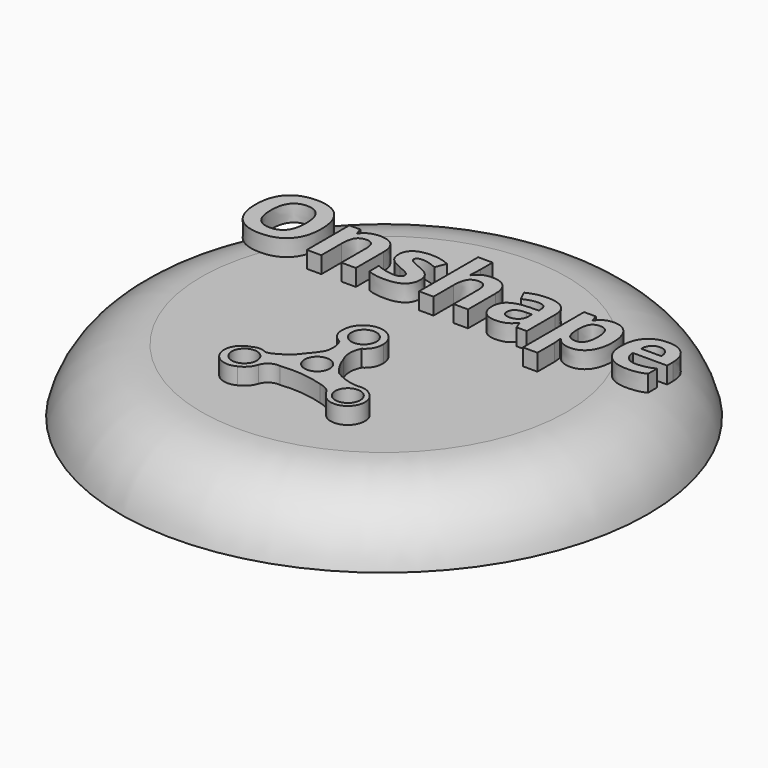
from build123d import *

# Parameters (mm, degrees)
F0_R         = 15.805
F1_DEPTH     = 3.81
F3_TEXT_SIZE = 5.8197312885
F4_DEPTH     = 1
F6_R         = 0.75
F7_DEPTH     = 1


# Not quite as in the source:
# - a fillet or chamfer that OpenCascade refuses, or shapes differently, is made with other operations: its cross-section is extruded or revolved along the edge and cut away or added
# - Text() gives the source's letters only with a copy of the font that has no kerning and outlines rounded to 1/6400 em; it was checked with that copy


with BuildPart() as f1:
    # F0 (on Top) → F1 (new body)
    with BuildSketch(Plane.XY):
        Circle(F0_R)
    extrude(amount=F1_DEPTH)

    # F2: fillet of radius 5 on 1 edges, made by hand

    # F2_s1 → F2_t2 (revolve, cut)
    with BuildSketch(Plane.XZ):
        with BuildLine():
            ThreePointArc((15.805, 0), (14.0349341008, 2.7438276526), (10.9486742284, 3.81))
            Line((10.9486742284, 3.81), (15.805, 3.81))
            Line((15.805, 3.81), (15.805, 0))
        make_face()
    revolve(axis=Axis((0, 0, 3.81), (0, 0, 1)), mode=Mode.SUBTRACT)

    # F3 (on face) → F4 (join)
    with BuildSketch(Plane.XY.offset(3.81)):
        with Locations((-12.6856137067, 3.719474189)):
            Text('Onshape', F3_TEXT_SIZE, font='Open Sans', font_style=FontStyle.BOLD, text_align=(TextAlign.LEFT, TextAlign.BOTTOM))
    extrude(amount=F4_DEPTH)

    # F6 (on face) → F7 (join)
    with BuildSketch(Plane.XY.offset(3.81)):
        with BuildLine():
            ThreePointArc((0.6517725415, -2.4959768634), (1.0496267958, -2.0753870693), (1.1650670785, -1.5080623617))
            ThreePointArc((1.1650670785, -1.5080623617), (-0.0326198642, -0.3425671333), (-1.230306807, -1.5080623617))
            ThreePointArc((-1.230306807, -1.5080623617), (-1.1063250132, -2.1233603441), (-0.6392406649, -2.5426398497))
            ThreePointArc((-0.6392406649, -2.5426398497), (-0.454048202, -3.1255160568), (-0.5286578089, -3.7325369194))
            ThreePointArc((-0.5286578089, -3.7325369194), (-0.8020989328, -4.1398712461), (-1.1165763717, -4.5164283365))
            ThreePointArc((-1.1165763717, -4.5164283365), (-1.5447835525, -5.0095430703), (-2.0964406431, -5.3591113538))
            ThreePointArc((-2.0964406431, -5.3591113538), (-2.3631101045, -5.5130095162), (-2.6647618506, -5.5746817961))
            ThreePointArc((-2.6647618506, -5.5746817961), (-3.0861033592, -5.455605353), (-3.5074448679, -5.5746817961))
            ThreePointArc((-3.5074448679, -5.5746817961), (-4.2369689218, -6.9676881184), (-2.7627481613, -7.5148125179))
            ThreePointArc((-2.7627481613, -7.5148125179), (-2.3440710579, -7.2189850446), (-2.0964406431, -6.7701158114))
            ThreePointArc((-2.0964406431, -6.7701158114), (-1.7679026827, -6.357753915), (-1.2537572766, -6.2409890816))
            ThreePointArc((-1.2537572766, -6.2409890816), (0.0722883441, -6.2340875096), (1.3722787844, -6.4957542345))
            ThreePointArc((1.3722787844, -6.4957542345), (1.6880765903, -6.6062751945), (1.9797945861, -6.7701158114))
            ThreePointArc((1.9797945861, -6.7701158114), (2.1665815655, -7.0510391049), (2.3717400618, -7.3188398965))
            ThreePointArc((2.3717400618, -7.3188398965), (3.9132771757, -7.2953405712), (3.6847579759, -5.7706544176))
            ThreePointArc((3.6847579759, -5.7706544176), (3.3163528533, -5.5785061448), (2.9008667916, -5.5746817961))
            ThreePointArc((2.9008667916, -5.5746817961), (2.1025476803, -5.4358737962), (1.3722787844, -5.0847493112))
            ThreePointArc((1.3722787844, -5.0847493112), (0.945670213, -4.5061587484), (0.6517725415, -3.8501205854))
            ThreePointArc((0.6517725415, -3.8501205854), (0.4894513603, -3.1730487244), (0.6517725415, -2.4959768634))
        make_face()
        with Locations((-3.1685938203, -6.4946736768)):
            Circle(F6_R, mode=Mode.SUBTRACT)
        with Locations((3.1130756933, -6.6076747296)):
            Circle(F6_R, mode=Mode.SUBTRACT)
        with Locations((0, -5.0080623617)):
            Circle(F6_R, mode=Mode.SUBTRACT)
        with Locations((0, -1.5080623617)):
            Circle(F6_R, mode=Mode.SUBTRACT)
    extrude(amount=F7_DEPTH)


solid = f1.part
